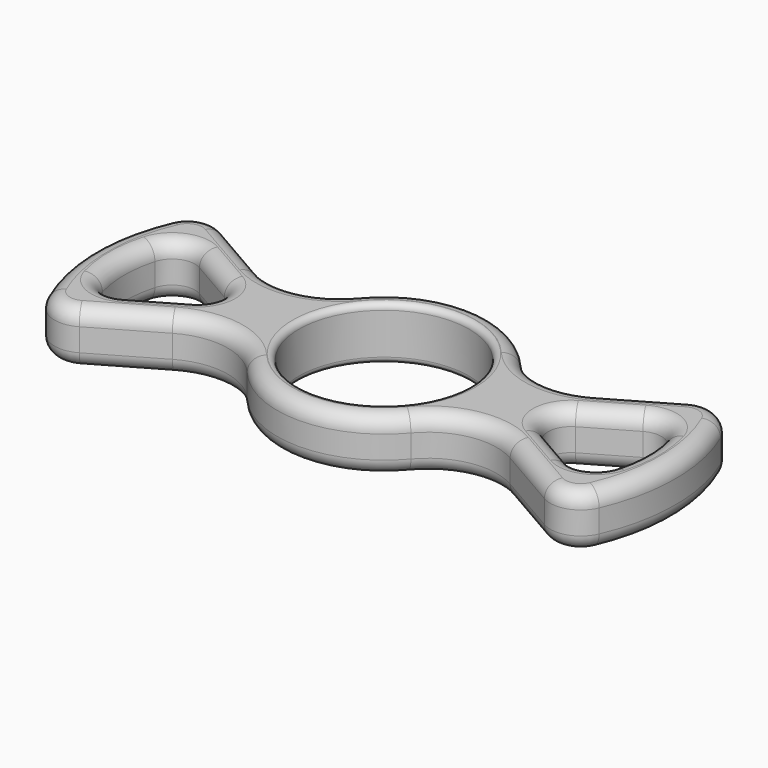
from build123d import *

# Parameters (mm, degrees)
F1_DEPTH = 7
F2_R     = 11.15
F3_DEPTH = 7.001
F4_R     = 9
F5_R     = 4
F7_DEPTH = 7.001
F8_R     = 3
F9_R     = 0.8
F10_R    = 2


with BuildPart() as f1:
    # F0 (on Top) → F1 (new body)
    with BuildSketch(Plane.XY):
        with BuildLine():
            Line((-34, -13.8564064606), (-13.8247516529, -2.2082213964))
            ThreePointArc((-13.8247516529, -2.2082213964), (0, -14), (13.8247516529, -2.2082213964))
            Line((13.8247516529, -2.2082213964), (34, -13.8564064606))
            ThreePointArc((34, -13.8564064606), (38.1913479533, 0), (34, 13.8564064606))
            Line((34, 13.8564064606), (13.8247516529, 2.2082213964))
            ThreePointArc((13.8247516529, 2.2082213964), (0, 14), (-13.8247516529, 2.2082213964))
            Line((-13.8247516529, 2.2082213964), (-34, 13.8564064606))
            ThreePointArc((-34, 13.8564064606), (-38.1913479533, 0), (-34, -13.8564064606))
        make_face()
    extrude(amount=F1_DEPTH)

    # F2 (on face) → F3 (cut, through all)
    with BuildSketch(Plane.XY.offset(7)):
        Circle(F2_R)
    extrude(amount=-F3_DEPTH, mode=Mode.SUBTRACT)

    # F4
    f4_edges = [f1.edges().sort_by_distance(p)[0] for p in [
        (-13.824752, -2.208221, 3.5),
        (13.824752, -2.208221, 3.5),
        (13.824752, 2.208221, 3.5),
        (-13.824752, 2.208221, 3.5),
    ]]
    fillet(f4_edges, radius=F4_R)

    # F5
    f5_edges = [f1.edges().sort_by_distance(p)[0] for p in [
        (-34, 13.856406, 3.5),
        (-34, -13.856406, 3.5),
        (34, 13.856406, 3.5),
        (34, -13.856406, 3.5),
    ]]
    fillet(f5_edges, radius=F5_R)

    # F6 (on face) → F7 (cut, through all)
    with BuildSketch(Plane.XY.offset(7)):
        with BuildLine():
            Line((-32, -7.7942286341), (-18.5, 0))
            Line((-18.5, 0), (-32, 7.7942286341))
            ThreePointArc((-32, 7.7942286341), (-34.0268113875, 0), (-32, -7.7942286341))
        make_face()
        with BuildLine():
            Line((32, 7.7942286341), (18.5, 0))
            Line((18.5, 0), (32, -7.7942286341))
            ThreePointArc((32, -7.7942286341), (34.0268113875, 0), (32, 7.7942286341))
        make_face()
    extrude(amount=-F7_DEPTH, mode=Mode.SUBTRACT)

    # F8
    f8_edges = [f1.edges().sort_by_distance(p)[0] for p in [
        (-18.5, 0, 3.5),
        (18.5, 0, 3.5),
        (-32, -7.794229, 3.5),
        (-32, 7.794229, 3.5),
        (32, 7.794229, 3.5),
        (32, -7.794229, 3.5),
    ]]
    fillet(f8_edges, radius=F8_R)

    # F9
    f9_edges = [f1.edges().sort_by_distance(p)[0] for p in [
        (-11.15, 0, 7),
        (11.15, 0, 3.5),
        (-11.15, 0, 0),
    ]]
    fillet(f9_edges, radius=F9_R)

    # F10
    f10_edges = [f1.edges().sort_by_distance(p)[0] for p in [
        (-11.95, 0, 7),
        (-34.026811, 0, 7),
        (-31.682853, 6.2698, 7),
        (-31.682853, -6.2698, 7),
        (-26.024465, 4.344252, 7),
        (-26.024465, -4.344252, 7),
        (-21.5, 0, 7),
        (-26.287749, 9.403736, 7),
        (-33.715572, 12.14673, 7),
        (-16.053404, 5.925373, 7),
        (-38.191348, 0, 7),
        (0, 14, 7),
        (-33.715572, -12.14673, 7),
        (16.053404, 5.925373, 7),
        (-26.287749, -9.403736, 7),
        (26.287749, 9.403736, 7),
        (-16.053404, -5.925373, 7),
        (33.715572, 12.14673, 7),
        (0, -14, 7),
        (38.191348, 0, 7),
        (16.053404, -5.925373, 7),
        (33.715572, -12.14673, 7),
        (26.287749, -9.403736, 7),
        (34.026811, 0, 7),
        (31.682853, -6.2698, 7),
        (31.682853, 6.2698, 7),
        (26.024465, -4.344252, 7),
        (26.024465, 4.344252, 7),
        (21.5, 0, 7),
        (-11.95, 0, 0),
        (-34.026811, 0, 0),
        (-31.682853, 6.2698, 0),
        (-31.682853, -6.2698, 0),
        (-26.024465, 4.344252, 0),
        (-26.024465, -4.344252, 0),
        (-21.5, 0, 0),
        (-26.287749, 9.403736, 0),
        (-33.715572, 12.14673, 0),
        (-16.053404, 5.925373, 0),
        (-38.191348, 0, 0),
        (0, 14, 0),
        (-33.715572, -12.14673, 0),
        (16.053404, 5.925373, 0),
        (-26.287749, -9.403736, 0),
        (26.287749, 9.403736, 0),
        (-16.053404, -5.925373, 0),
        (33.715572, 12.14673, 0),
        (0, -14, 0),
        (38.191348, 0, 0),
        (16.053404, -5.925373, 0),
        (33.715572, -12.14673, 0),
        (26.287749, -9.403736, 0),
        (34.026811, 0, 0),
        (31.682853, -6.2698, 0),
        (31.682853, 6.2698, 0),
        (26.024465, -4.344252, 0),
        (26.024465, 4.344252, 0),
        (21.5, 0, 0),
    ]]
    fillet(f10_edges, radius=F10_R)


solid = f1.part
